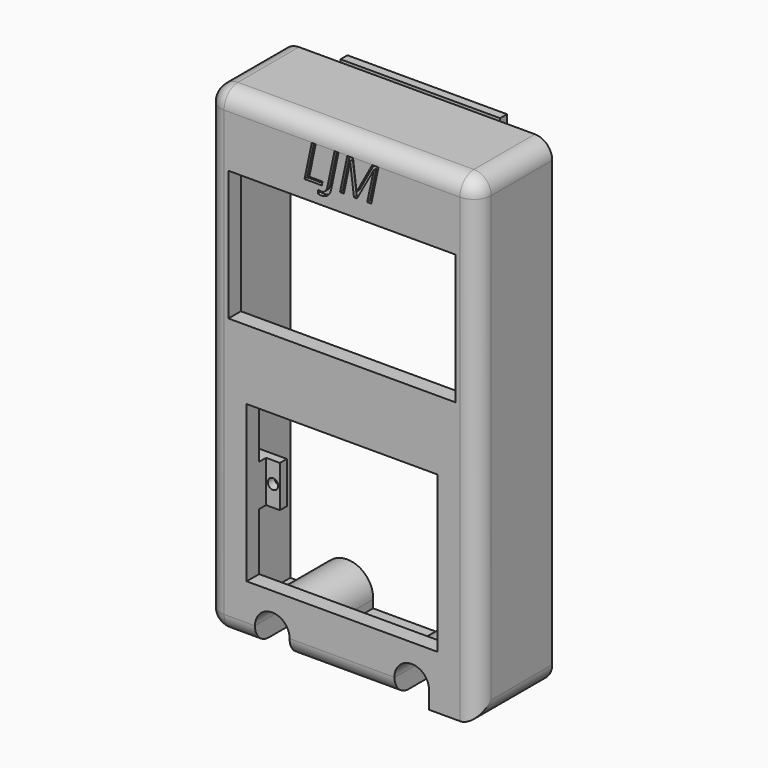
from build123d import *

# Parameters (mm, degrees)
F0_W         = 55
F0_H         = 45
F0_W_2       = 65.5
F0_H_2       = 37.5
F0_R         = 2
F1_DEPTH     = 27
F2_W         = 46
F2_H         = 2.5
F3_DEPTH     = 3.7
F2_W_2       = 55
F2_H_2       = 45
F2_W_3       = 65.5
F2_H_3       = 37.5
F0_W_3       = 46
F0_H_3       = 8
F4_DEPTH     = 22.5
F5_DEPTH     = 20
F6_R         = 5
F7_TEXT_SIZE = 13.847478355
F8_DEPTH     = 1
F9_W         = 46
F9_H         = 2.5
F10_DEPTH    = 11
F11_W        = 9
F11_H        = 12
F11_W_2      = 4
F11_R        = 1.5
F12_DEPTH    = 5
F13_DEPTH    = 2.5


# Not quite as in the source:
# - Text() gives the source's letters only with a copy of the font that has no kerning and outlines rounded to 1/6400 em; it was checked with that copy


with BuildPart() as f1:
    # F0 (on Front) → F1 (new body)
    with BuildSketch(Plane.XZ):
        with BuildLine():
            Line((39, -69), (39, 69))
            Line((39, 69), (23, 69))
            Line((23, 69), (-23, 69))
            Line((-23, 69), (-39, 69))
            Line((-39, 69), (-39, -69))
            Line((-39, -69), (-27.6, -69))
            Line((-27.6, -69), (-27.6, -64))
            ThreePointArc((-27.6, -64), (-20.0246777515, -56.5003782389), (-12.6015129176, -64.1506368998))
            Line((-12.6015129176, -64.1506368998), (-12.6989316389, -69))
            Line((-12.6989316389, -69), (12.6989316389, -69))
            Line((12.6989316389, -69), (12.6015129176, -64.1506368998))
            ThreePointArc((12.6015129176, -64.1506368998), (20.0246777515, -56.5003782389), (27.6, -64))
            Line((27.6, -64), (27.6, -69))
            Line((27.6, -69), (39, -69))
        make_face()
        with Locations((0, -31)):
            Rectangle(F0_W, F0_H, mode=Mode.SUBTRACT)
        with Locations((0, 30.25)):
            Rectangle(F0_W_2, F0_H_2, mode=Mode.SUBTRACT)
        with BuildLine():
            Line((15.1994360466, -69), (25.1, -69))
            Line((25.1, -69), (25.1, -64))
            ThreePointArc((25.1, -64), (20.0497851677, -59.0002521593), (15.1010086118, -64.1004245998))
            Line((15.1010086118, -64.1004245998), (15.1994360466, -69))
        make_face()
        with Locations((20.1, -64)):
            Circle(F0_R, mode=Mode.SUBTRACT)
        with BuildLine():
            Line((-25.1, -64), (-25.1, -69))
            Line((-25.1, -69), (-15.1994360466, -69))
            Line((-15.1994360466, -69), (-15.1010086118, -64.1004245998))
            ThreePointArc((-15.1010086118, -64.1004245998), (-20.0497851677, -59.0002521593), (-25.1, -64))
        make_face()
        with Locations((-20.1, -64)):
            Circle(F0_R, mode=Mode.SUBTRACT)
        with BuildLine():
            Line((25.1, -69), (27.6, -69))
            Line((27.6, -69), (27.6, -64))
            ThreePointArc((27.6, -64), (20.0246777515, -56.5003782389), (12.6015129176, -64.1506368998))
            Line((12.6015129176, -64.1506368998), (12.6989316389, -69))
            Line((12.6989316389, -69), (15.1994360466, -69))
            Line((15.1994360466, -69), (15.1010086118, -64.1004245998))
            ThreePointArc((15.1010086118, -64.1004245998), (20.0497851677, -59.0002521593), (25.1, -64))
            Line((25.1, -64), (25.1, -69))
        make_face()
        with BuildLine():
            Line((-27.6, -64), (-27.6, -69))
            Line((-27.6, -69), (-25.1, -69))
            Line((-25.1, -69), (-25.1, -64))
            ThreePointArc((-25.1, -64), (-20.0497851677, -59.0002521593), (-15.1010086118, -64.1004245998))
            Line((-15.1010086118, -64.1004245998), (-15.1994360466, -69))
            Line((-15.1994360466, -69), (-12.6989316389, -69))
            Line((-12.6989316389, -69), (-12.6015129176, -64.1506368998))
            ThreePointArc((-12.6015129176, -64.1506368998), (-20.0246777515, -56.5003782389), (-27.6, -64))
        make_face()
    extrude(amount=-F1_DEPTH)

    # F2 (on face) → F3 (join)
    with BuildSketch(Plane(origin=(0, 27, 0), x_dir=(-1, 0, 0), z_dir=(0, 1, 0))):
        with Locations((0, 56.75)):
            Rectangle(F2_W, F2_H)
    extrude(amount=F3_DEPTH)

    # F2 (on face) + F0 (on Front) → F4 (cut)
    with BuildSketch(Plane(origin=(0, 27, 0), x_dir=(-1, 0, 0), z_dir=(0, 1, 0))):
        with BuildLine():
            Line((-23, 58), (-23, 66.5))
            Line((-23, 66.5), (-36.5, 66.5))
            Line((-36.5, 66.5), (-36.5, -66.5))
            Line((-36.5, -66.5), (-27.6000034064, -66.5))
            Line((-27.6000034064, -66.5), (-27.6000034064, -64))
            ThreePointArc((-27.6000034064, -64), (-20.0246811579, -56.5003782389), (-12.601516324, -64.1506368998))
            Line((-12.601516324, -64.1506368998), (-12.6487126144, -66.5))
            Line((-12.6487126144, -66.5), (12.648709208, -66.5))
            Line((12.648709208, -66.5), (12.6015129176, -64.1506368998))
            ThreePointArc((12.6015129176, -64.1506368998), (20.0246777515, -56.5003782389), (27.6, -64))
            Line((27.6, -64), (27.6, -66.5))
            Line((27.6, -66.5), (36.5, -66.5))
            Line((36.5, -66.5), (36.5, 66.5))
            Line((36.5, 66.5), (23, 66.5))
            Line((23, 66.5), (23, 58))
            Line((23, 58), (23, 55.5))
            Line((23, 55.5), (-23, 55.5))
            Line((-23, 55.5), (-23, 58))
        make_face()
        with Locations((0, -31)):
            Rectangle(F2_W_2, F2_H_2, mode=Mode.SUBTRACT)
        with Locations((0, 30.25)):
            Rectangle(F2_W_3, F2_H_3, mode=Mode.SUBTRACT)
    with BuildSketch(Plane.XZ):
        with BuildLine():
            Line((39, -69), (39, 69))
            Line((39, 69), (23, 69))
            Line((23, 69), (-23, 69))
            Line((-23, 69), (-39, 69))
            Line((-39, 69), (-39, -69))
            Line((-39, -69), (-27.6, -69))
            Line((-27.6, -69), (-27.6, -64))
            ThreePointArc((-27.6, -64), (-20.0246777515, -56.5003782389), (-12.6015129176, -64.1506368998))
            Line((-12.6015129176, -64.1506368998), (-12.6989316389, -69))
            Line((-12.6989316389, -69), (12.6989316389, -69))
            Line((12.6989316389, -69), (12.6015129176, -64.1506368998))
            ThreePointArc((12.6015129176, -64.1506368998), (20.0246777515, -56.5003782389), (27.6, -64))
            Line((27.6, -64), (27.6, -69))
            Line((27.6, -69), (39, -69))
        make_face()
        with Locations((0, -31)):
            Rectangle(F0_W, F0_H, mode=Mode.SUBTRACT)
        with Locations((0, 30.25)):
            Rectangle(F0_W_2, F0_H_2, mode=Mode.SUBTRACT)
        with Locations((0, 73)):
            Rectangle(F0_W_3, F0_H_3)
        with BuildLine():
            Line((25.1, -69), (27.6, -69))
            Line((27.6, -69), (27.6, -64))
            ThreePointArc((27.6, -64), (20.0246777515, -56.5003782389), (12.6015129176, -64.1506368998))
            Line((12.6015129176, -64.1506368998), (12.6989316389, -69))
            Line((12.6989316389, -69), (15.1994360466, -69))
            Line((15.1994360466, -69), (15.1010086118, -64.1004245998))
            ThreePointArc((15.1010086118, -64.1004245998), (20.0497851677, -59.0002521593), (25.1, -64))
            Line((25.1, -64), (25.1, -69))
        make_face()
        with BuildLine():
            Line((15.1994360466, -69), (25.1, -69))
            Line((25.1, -69), (25.1, -64))
            ThreePointArc((25.1, -64), (20.0497851677, -59.0002521593), (15.1010086118, -64.1004245998))
            Line((15.1010086118, -64.1004245998), (15.1994360466, -69))
        make_face()
        with Locations((20.1, -64)):
            Circle(F0_R, mode=Mode.SUBTRACT)
        with BuildLine():
            Line((-27.6, -64), (-27.6, -69))
            Line((-27.6, -69), (-25.1, -69))
            Line((-25.1, -69), (-25.1, -64))
            ThreePointArc((-25.1, -64), (-20.0497851677, -59.0002521593), (-15.1010086118, -64.1004245998))
            Line((-15.1010086118, -64.1004245998), (-15.1994360466, -69))
            Line((-15.1994360466, -69), (-12.6989316389, -69))
            Line((-12.6989316389, -69), (-12.6015129176, -64.1506368998))
            ThreePointArc((-12.6015129176, -64.1506368998), (-20.0246777515, -56.5003782389), (-27.6, -64))
        make_face()
        with BuildLine():
            Line((-25.1, -64), (-25.1, -69))
            Line((-25.1, -69), (-15.1994360466, -69))
            Line((-15.1994360466, -69), (-15.1010086118, -64.1004245998))
            ThreePointArc((-15.1010086118, -64.1004245998), (-20.0497851677, -59.0002521593), (-25.1, -64))
        make_face()
        with Locations((-20.1, -64)):
            Circle(F0_R, mode=Mode.SUBTRACT)
    extrude(amount=-F4_DEPTH, dir=(0, 1, 0), mode=Mode.SUBTRACT)

    # F0 (on Front) → F5 (cut)
    with BuildSketch(Plane.XZ):
        with BuildLine():
            Line((-25.1, -64), (-25.1, -69))
            Line((-25.1, -69), (-15.1994360466, -69))
            Line((-15.1994360466, -69), (-15.1010086118, -64.1004245998))
            ThreePointArc((-15.1010086118, -64.1004245998), (-20.0497851677, -59.0002521593), (-25.1, -64))
        make_face()
        with Locations((-20.1, -64)):
            Circle(F0_R, mode=Mode.SUBTRACT)
        with BuildLine():
            Line((15.1994360466, -69), (25.1, -69))
            Line((25.1, -69), (25.1, -64))
            ThreePointArc((25.1, -64), (20.0497851677, -59.0002521593), (15.1010086118, -64.1004245998))
            Line((15.1010086118, -64.1004245998), (15.1994360466, -69))
        make_face()
        with Locations((20.1, -64)):
            Circle(F0_R, mode=Mode.SUBTRACT)
    extrude(amount=-F5_DEPTH, mode=Mode.SUBTRACT)

    # F6
    f6_edges = [f1.edges().sort_by_distance(p)[0] for p in [
        (39, 13.5, 69),
        (39, 0, 0),
        (0, 0, 69),
        (-39, 0, 0),
        (-32.05, 0, -69),
        (0, 0, -69),
        (39, 13.5, -69),
        (-39, 13.5, -69),
        (-39, 13.5, 69),
    ]]
    fillet(f6_edges, radius=F6_R)

    # F7 (on face) → F8 (cut)
    with BuildSketch(Plane.XZ):
        with Locations((-11.3949601182, 54.0298155844)):
            Text('LJM', F7_TEXT_SIZE, font='Open Sans', font_style=FontStyle.ITALIC, text_align=(TextAlign.LEFT, TextAlign.BOTTOM))
    extrude(amount=-F8_DEPTH, mode=Mode.SUBTRACT)

    # F9 (on face) → F10 (join, through all)
    with BuildSketch(Plane.XY.offset(58)):
        with Locations((0, 29.45)):
            Rectangle(F9_W, F9_H)
    extrude(amount=F10_DEPTH)

    # F11 (on face) → F12 (join)
    with BuildSketch(Plane(origin=(0, 4.5, 0), x_dir=(-1, 0, 0), z_dir=(0, 1, 0))):
        with Locations((-32, -31)):
            Rectangle(F11_W, F11_H)
        with Locations((-25.5, -31)):
            Rectangle(F11_W_2, F11_H)
        with Locations((-25.5, -31)):
            Circle(F11_R, mode=Mode.SUBTRACT)
        with Locations((25.5, -31)):
            Rectangle(F11_W_2, F11_H)
        with Locations((25.5, -31)):
            Circle(F11_R, mode=Mode.SUBTRACT)
        with Locations((32, -31)):
            Rectangle(F11_W, F11_H)
    extrude(amount=F12_DEPTH)

    # F13 (cut): faces of the model
    f13_faces = [f1.faces().sort_by_distance(p)[0] for p in [
        (-25.5, 4.5, -25.1264911064),
        (25.5, 4.5, -25.1264911064),
    ]]
    extrude(f13_faces, amount=-F13_DEPTH, mode=Mode.SUBTRACT)


solid = f1.part
